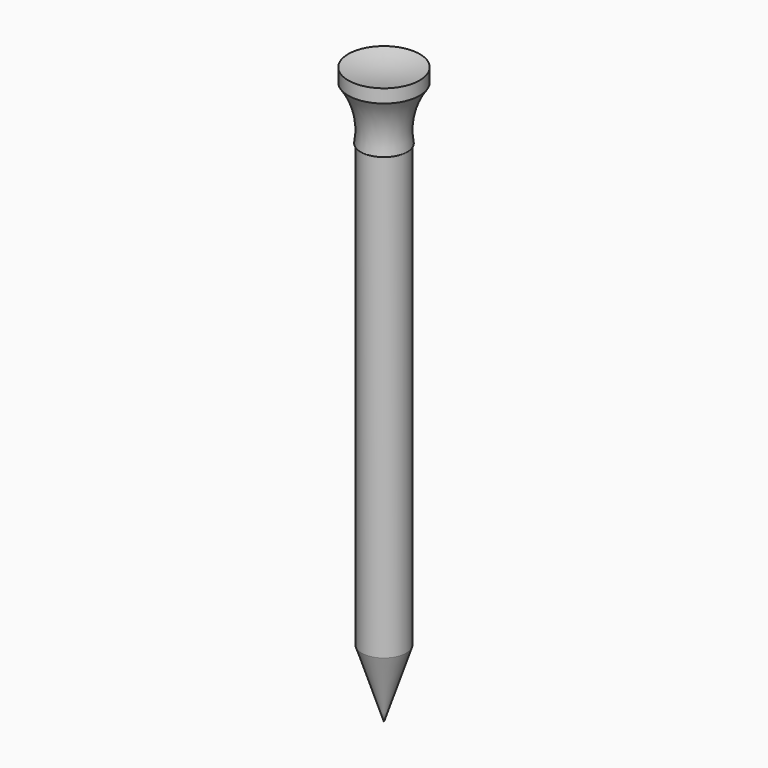
from build123d import *


# Not quite as in the source:
# - a feature names something its author has since deleted; it is built from what else it names


with BuildPart() as f1:
    # F0 (on Front) → F1 (revolve)
    with BuildSketch(Plane.XZ):
        Polygon((0, -62.7388355625), (0, 0), (-3.175, 0), (-3.175, -62.7388355625), (0, -72.39), align=None)
    revolve(axis=Axis((0, 0, -31.3694177812), (0, 0, -1)))

    # F2 (on Front) → F3 (revolve)
    with BuildSketch(Plane.XZ):
        with BuildLine():
            ThreePointArc((-5.08, 7.62), (-3.4362663376, 3.9863656813), (-3.3177447348, 0))
            Line((-3.3177447348, 0), (0, 0))
            Line((0, 0), (0, 7.62))
            Line((0, 7.62), (-5.08, 7.62))
        make_face()
        with BuildLine():
            Line((-5.08, 9.525), (-5.08, 7.62))
            Line((-5.08, 7.62), (0, 7.62))
            Line((0, 7.62), (0, 8.8351770144))
            ThreePointArc((0, 8.8351770144), (-2.5633111278, 9.0084205117), (-5.08, 9.525))
        make_face()
    revolve(axis=Axis((0, 0, 8.2275885072), (0, 0, 1)))


solid = f1.part
